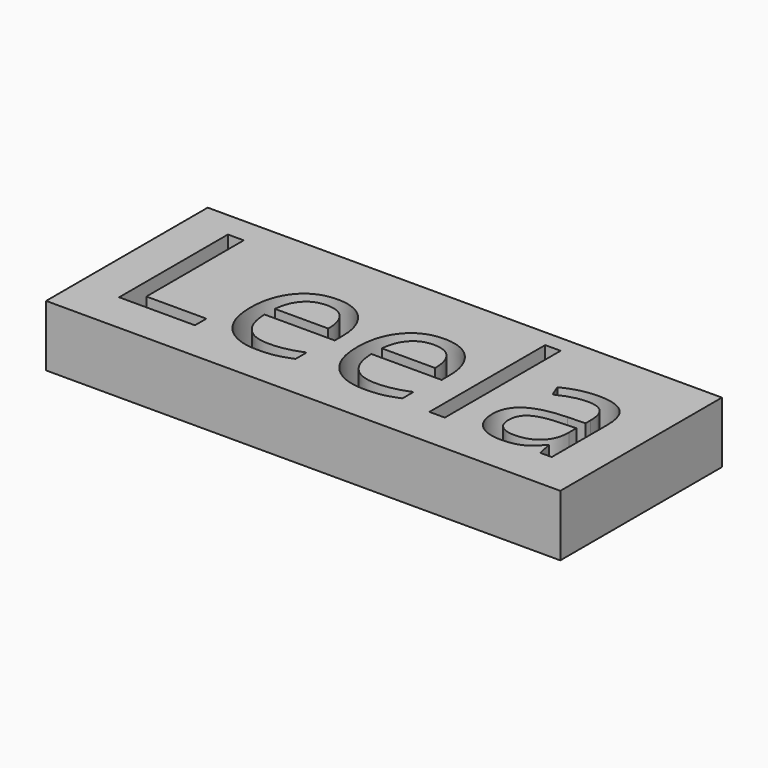
from build123d import *

# Parameters (mm, degrees)
F0_W         = 64.0079975128
F0_H         = 25.1460019499
F1_DEPTH     = 7.62
F2_TEXT_SIZE = 23.7066680307
F3_DEPTH     = 7.621


# Not quite as in the source:
# - Text() gives the source's letters only with a copy of the font that has no kerning and outlines rounded to 1/6400 em; it was checked with that copy


with BuildPart() as f1:
    # F0 (on Top) → F1 (new body)
    with BuildSketch(Plane.XY):
        with Locations((32.0039987564, 12.573000975)):
            Rectangle(F0_W, F0_H)
    extrude(amount=F1_DEPTH)

    # F2 (on face) → F3 (cut, through all)
    with BuildSketch(Plane.XY.offset(7.62)):
        with Locations((2.7432027273, 5.0292001106)):
            Text('Leela', F2_TEXT_SIZE, font='Open Sans', text_align=(TextAlign.LEFT, TextAlign.BOTTOM))
    extrude(amount=-F3_DEPTH, mode=Mode.SUBTRACT)


solid = f1.part
